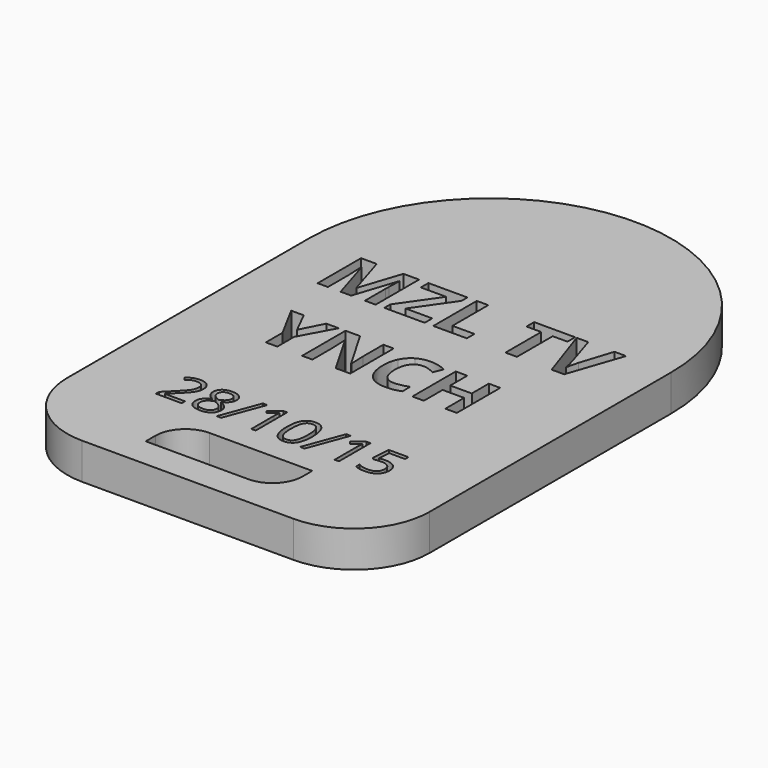
from build123d import *

# Parameters (mm, degrees)
F1_DEPTH     = 2.4
F3_TEXT_SIZE = 3.6521342159
F4_DEPTH     = 25
F6_DEPTH     = 25


# Not quite as in the source:
# - Text() gives the source's letters only with a copy of the font that has no kerning and outlines rounded to 1/6400 em; it was checked with that copy


with BuildPart() as f1:
    # F0 (on Top) → F1 (new body)
    with BuildSketch(Plane.XY):
        with BuildLine():
            Line((12, -20), (12, 0))
            ThreePointArc((12, 0), (0, 12), (-12, 0))
            Line((-12, 0), (-12, -20))
            ThreePointArc((-12, -20), (-10.5355339059, -23.5355339059), (-7, -25))
            Line((-7, -25), (7, -25))
            ThreePointArc((7, -25), (10.5355339059, -23.5355339059), (12, -20))
        make_face()
        Polygon((-6.8321467114, -6.8770319874), (-6.0872594539, -8.3565810173), (-5.3376527418, -6.8770319874), (-4.5164676343, -6.8770319874), (-5.7089165069, -9.0723649712), (-5.7089165069, -10.4708966964), (-6.4656024009, -10.4708966964), (-6.4656024009, -9.0967488201), (-7.6580512735, -6.8770319874), align=None, mode=Mode.SUBTRACT)
        with BuildLine():
            Line((-0.8761949547, -6.8770319874), (-0.8761949547, -10.4708966964))
            Line((-0.8761949547, -10.4708966964), (-1.8444697318, -10.4708966964))
            Line((-1.8444697318, -10.4708966964), (-3.4081823695, -7.7524908233))
            Line((-3.4081823695, -7.7524908233), (-3.4302064911, -7.7524908233))
            add(Edge.make_bspline(
                [(-3.4302064911, -7.7524908233), (-3.3830119447, -8.472207656), (-3.3830119447, -8.7797587834)],
                knots=[0, 0, 0, 1, 1, 1], degree=2))
            Line((-3.3830119447, -8.7797587834), (-3.3830119447, -10.4708966964))
            Line((-3.3830119447, -10.4708966964), (-4.0641865646, -10.4708966964))
            Line((-4.0641865646, -10.4708966964), (-4.0641865646, -6.8770319874))
            Line((-4.0641865646, -6.8770319874), (-3.1029909694, -6.8770319874))
            Line((-3.1029909694, -6.8770319874), (-1.5424246348, -9.5686942842))
            Line((-1.5424246348, -9.5686942842), (-1.5251199678, -9.5686942842))
            add(Edge.make_bspline(
                [(-1.5251199678, -9.5686942842), (-1.5620890292, -8.8678552701), (-1.5620890292, -8.5783953854)],
                knots=[0, 0, 0, 1, 1, 1], degree=2))
            Line((-1.5620890292, -8.5783953854), (-1.5620890292, -6.8770319874))
            Line((-1.5620890292, -6.8770319874), (-0.8761949547, -6.8770319874))
        make_face(mode=Mode.SUBTRACT)
        with BuildLine():
            add(Edge.make_bspline(
                [(1.9554778298, -7.5310697431), (1.7517547045, -7.4598846356), (1.5551107611, -7.4598846356)],
                knots=[0, 0, 0, 1, 1, 1], degree=2))
            add(Edge.make_bspline(
                [(1.5551107611, -7.4598846356), (1.124853813, -7.4598846356), (0.888881081, -7.7831672784)],
                knots=[0, 0, 0, 1, 1, 1], degree=2))
            add(Edge.make_bspline(
                [(0.888881081, -7.7831672784), (0.6529083489, -8.1064499213), (0.6529083489, -8.6837965391)],
                knots=[0, 0, 0, 1, 1, 1], degree=2))
            add(Edge.make_bspline(
                [(0.6529083489, -8.6837965391), (0.6529083489, -9.8856843209), (1.5551107611, -9.8856843209)],
                knots=[0, 0, 0, 1, 1, 1], degree=2))
            add(Edge.make_bspline(
                [(1.5551107611, -9.8856843209), (1.9334537081, -9.8856843209), (2.4714715372, -9.6969061353)],
                knots=[0, 0, 0, 1, 1, 1], degree=2))
            Line((2.4714715372, -9.6969061353), (2.4714715372, -10.3356056633))
            add(Edge.make_bspline(
                [(2.4714715372, -10.3356056633), (2.0294159525, -10.5204509701), (1.4835323657, -10.5204509701)],
                knots=[0, 0, 0, 1, 1, 1], degree=2))
            add(Edge.make_bspline(
                [(1.4835323657, -10.5204509701), (0.6993163196, -10.5204509701), (0.2840043112, -10.0445726272)],
                knots=[0, 0, 0, 1, 1, 1], degree=2))
            add(Edge.make_bspline(
                [(0.2840043112, -10.0445726272), (-0.1313076972, -9.5686942842), (-0.1313076972, -8.6790770844)],
                knots=[0, 0, 0, 1, 1, 1], degree=2))
            add(Edge.make_bspline(
                [(-0.1313076972, -8.6790770844), (-0.1313076972, -8.1182485579), (0.072808716, -7.6966439434)],
                knots=[0, 0, 0, 1, 1, 1], degree=2))
            add(Edge.make_bspline(
                [(0.072808716, -7.6966439434), (0.2769251292, -7.2750393288), (0.6592009551, -7.0504719455)],
                knots=[0, 0, 0, 1, 1, 1], degree=2))
            add(Edge.make_bspline(
                [(0.6592009551, -7.0504719455), (1.041476781, -6.8259045621), (1.5551107611, -6.8259045621)],
                knots=[0, 0, 0, 1, 1, 1], degree=2))
            add(Edge.make_bspline(
                [(1.5551107611, -6.8259045621), (2.0781836504, -6.8259045621), (2.6067625702, -7.0783953854)],
                knots=[0, 0, 0, 1, 1, 1], degree=2))
            Line((2.6067625702, -7.0783953854), (2.3613509289, -7.6982170949))
            add(Edge.make_bspline(
                [(2.3613509289, -7.6982170949), (2.1592009551, -7.6022548506), (1.9554778298, -7.5310697431)],
                knots=[0, 0, 0, 1, 1, 1], degree=2))
        make_face(mode=Mode.SUBTRACT)
        Polygon((6.1809628848, -6.8770319874), (6.1809628848, -10.4708966964), (5.4211306877, -10.4708966964), (5.4211306877, -8.9197692711), (3.9982151135, -8.9197692711), (3.9982151135, -10.4708966964), (3.236023189, -10.4708966964), (3.236023189, -6.8770319874), (3.9982151135, -6.8770319874), (3.9982151135, -8.2857891977), (5.4211306877, -8.2857891977), (5.4211306877, -6.8770319874), align=None, mode=Mode.SUBTRACT)
        with BuildLine():
            Line((-6.2941288823, -3.6245411641), (-6.9926081692, -3.6245411641))
            Line((-6.9926081692, -3.6245411641), (-7.85784152, -0.805453592))
            Line((-7.85784152, -0.805453592), (-7.8798656416, -0.805453592))
            add(Edge.make_bspline(
                [(-7.8798656416, -0.805453592), (-7.8326710952, -1.6651809124), (-7.8326710952, -1.9530676455)],
                knots=[0, 0, 0, 1, 1, 1], degree=2))
            Line((-7.8326710952, -1.9530676455), (-7.8326710952, -3.6245411641))
            Line((-7.8326710952, -3.6245411641), (-8.5138457151, -3.6245411641))
            Line((-8.5138457151, -3.6245411641), (-8.5138457151, -0.0306764552))
            Line((-8.5138457151, -0.0306764552), (-7.4763522699, -0.0306764552))
            Line((-7.4763522699, -0.0306764552), (-6.6260638587, -2.7789722077))
            Line((-6.6260638587, -2.7789722077), (-6.611118919, -2.7789722077))
            Line((-6.611118919, -2.7789722077), (-5.7089165069, -0.0306764552))
            Line((-5.7089165069, -0.0306764552), (-4.6722096374, -0.0306764552))
            Line((-4.6722096374, -0.0306764552), (-4.6722096374, -3.6245411641))
            Line((-4.6722096374, -3.6245411641), (-5.3824875609, -3.6245411641))
            Line((-5.3824875609, -3.6245411641), (-5.3824875609, -1.9231777661))
            add(Edge.make_bspline(
                [(-5.3824875609, -1.9231777661), (-5.3824875609, -1.8028316728), (-5.378554682, -1.6455165181)],
                knots=[0, 0, 0, 1, 1, 1], degree=2))
            add(Edge.make_bspline(
                [(-5.378554682, -1.6455165181), (-5.3746218032, -1.4882013634), (-5.3455184995, -0.8101730467)],
                knots=[0, 0, 0, 1, 1, 1], degree=2))
            Line((-5.3455184995, -0.8101730467), (-5.3675426212, -0.8101730467))
            Line((-5.3675426212, -0.8101730467), (-6.2941288823, -3.6245411641))
        make_face(mode=Mode.SUBTRACT)
        Polygon((-1.4252248446, -2.9952805454), (-1.4252248446, -3.6245411641), (-4.0995824744, -3.6245411641), (-4.0995824744, -3.1305715784), (-2.3761949547, -0.6599370739), (-4.052387928, -0.6599370739), (-4.052387928, -0.0306764552), (-1.4716328152, -0.0306764552), (-1.4716328152, -0.5222863136), (-3.1926606076, -2.9952805454), align=None, mode=Mode.SUBTRACT)
        Polygon((1.3671191512, -3.6245411641), (-0.8525976815, -3.6245411641), (-0.8525976815, -0.0306764552), (-0.090405757, -0.0306764552), (-0.090405757, -2.9952805454), (1.3671191512, -2.9952805454), align=None, mode=Mode.SUBTRACT)
        Polygon((4.6864689153, -0.6646565286), (4.6864689153, -3.6245411641), (3.9242769908, -3.6245411641), (3.9242769908, -0.6646565286), (2.9481364559, -0.6646565286), (2.9481364559, -0.0306764552), (5.6618228744, -0.0306764552), (5.6618228744, -0.6646565286), align=None, mode=Mode.SUBTRACT)
        with BuildLine():
            Line((7.5842140647, -2.1693759832), (8.2646021088, -0.0306764552))
            Line((8.2646021088, -0.0306764552), (9.0338732152, -0.0306764552))
            Line((9.0338732152, -0.0306764552), (7.812321039, -3.6245411641))
            Line((7.812321039, -3.6245411641), (6.9816970222, -3.6245411641))
            Line((6.9816970222, -3.6245411641), (5.7625045734, -0.0306764552))
            Line((5.7625045734, -0.0306764552), (6.5317756798, -0.0306764552))
            Line((6.5317756798, -0.0306764552), (7.208230845, -2.1693759832))
            add(Edge.make_bspline(
                [(7.208230845, -2.1693759832), (7.2640777249, -2.3589407446), (7.3246440595, -2.6106449921)],
                knots=[0, 0, 0, 1, 1, 1], degree=2))
            add(Edge.make_bspline(
                [(7.3246440595, -2.6106449921), (7.385210394, -2.8623492396), (7.3993687579, -2.9606712113)],
                knots=[0, 0, 0, 1, 1, 1], degree=2))
            add(Edge.make_bspline(
                [(7.3993687579, -2.9606712113), (7.42689891, -2.7349239643), (7.5842140647, -2.1693759832)],
                knots=[0, 0, 0, 1, 1, 1], degree=2))
        make_face(mode=Mode.SUBTRACT)
    extrude(amount=F1_DEPTH)

    # F3 (on face) → F4 (cut)
    with BuildSketch(Plane.XY.offset(2.4)):
        with Locations((-7.5, -18.5085221499)):
            Text('28/10/15', F3_TEXT_SIZE, font='Open Sans', text_align=(TextAlign.LEFT, TextAlign.BOTTOM))
    extrude(amount=-F4_DEPTH, mode=Mode.SUBTRACT)

    # F5 (on face) → F6 (cut)
    with BuildSketch(Plane.XY.offset(2.4)):
        with BuildLine():
            Line((4.3968013488, -21), (4.3968013488, -20.2095601261))
            Line((4.3968013488, -20.2095601261), (-2.3968013488, -20.2095601261))
            ThreePointArc((-2.3968013488, -20.2095601261), (-3.8110149111, -20.7953465637), (-4.3968013488, -22.2095601261))
            Line((-4.3968013488, -22.2095601261), (-4.3968013488, -23))
            Line((-4.3968013488, -23), (2.3968013488, -23))
            ThreePointArc((2.3968013488, -23), (3.8110149111, -22.4142135624), (4.3968013488, -21))
        make_face()
    extrude(amount=-F6_DEPTH, mode=Mode.SUBTRACT)


solid = f1.part
